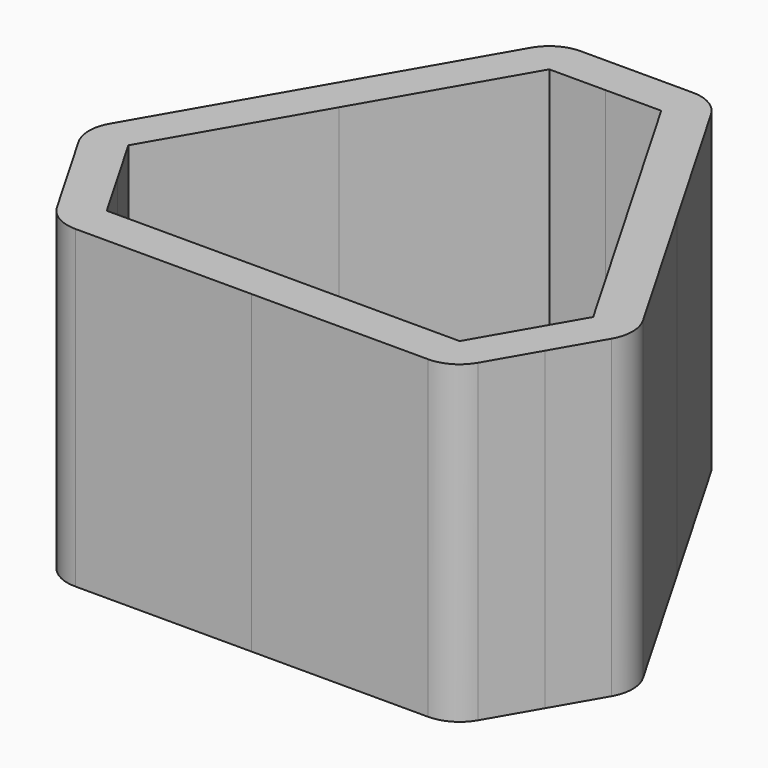
from build123d import *

# Parameters (mm, degrees)
F1_DEPTH = 50.8
F2_R     = 6.35
F3_T     = 6.35
F6_COUNT = 3


# Not quite as in the source:
# - a shell that OpenCascade refuses in one call is made with other operations: the cavity is built on its own and cut out


with BuildPart() as f1:
    # F0 (on Top) → F1 (new body)
    with BuildSketch(Plane.XY):
        Polygon((0, 44.4439283112), (0, 0), (28.7697854807, 16.6102433918), (12.7, 44.4439283112), align=None)
    extrude(amount=F1_DEPTH)

    # F2
    f2_edges = [f1.edges().sort_by_distance(p)[0] for p in [
        (12.7, 44.443928, 25.4),
    ]]
    fillet(f2_edges, radius=F2_R)

    # F3: shell of thickness 6.35, made by hand


with BuildPart() as f3_core1:
    # F3_t2: copy of F1
    add(f1.part)

    # the walls: a layer under each face that stays
    f3_faces = [f3_core1.faces().sort_by_distance(p)[0] for p in [
        (21.6514362927, 28.9395858515, 25.4),
        (4.5169128953, 44.4439283112, 25.4),
    ]]
    thicken(f3_faces, amount=-F3_T, mode=Mode.SUBTRACT)


with BuildPart() as f1_1:
    add(f1.part)

    # what is left inside the walls is the cavity
    f3_cavity = [f3_core1.part.solids().sort_by_distance(p)[0] for p in [
        (0.0635, 19.046964, 33.866667),
    ]]
    add(f3_cavity, mode=Mode.SUBTRACT)

    # F4: F1 across face


with BuildPart() as f1_2:
    add(f1_1.part)
    add(f1_1.part.mirror(Plane(origin=(26.0201548237, 15.0227433918, 25.4), x_dir=(0.8660254038, 0.5, 0), z_dir=(0.5, -0.8660254038, 0))))

    # F6: F1 ×3 about axis
    f6_axis = Axis((0, 0, 37.9905737936), (0, 0, -1))


with BuildPart() as f1_3:
    add(f1_2.part)
    for i in range(1, F6_COUNT):
        add(f1_2.part.rotate(f6_axis, i * 360 / F6_COUNT))


solid = f1_3.part
